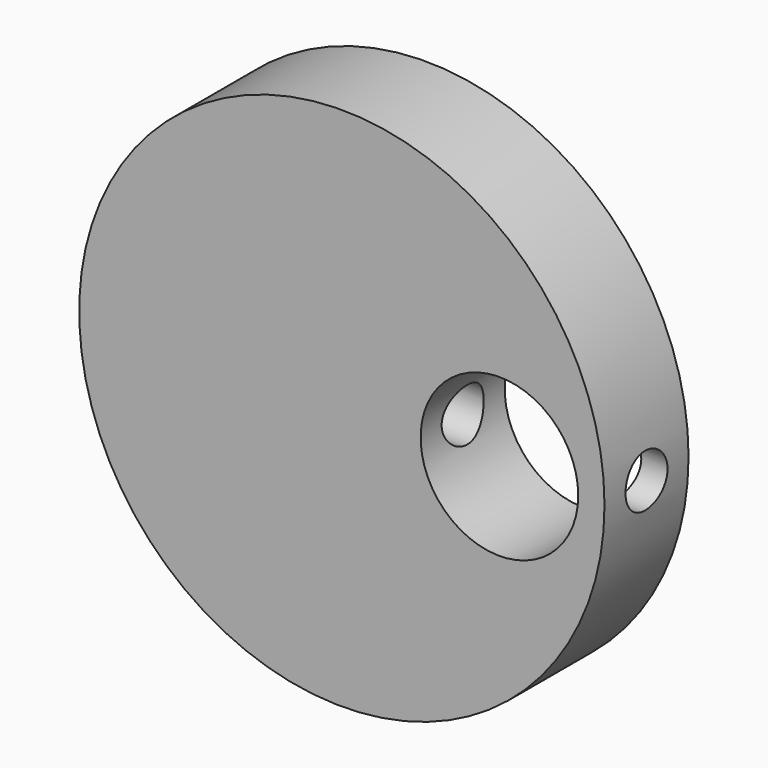
from build123d import *

# Parameters (mm, degrees)
F0_R     = 15.875
F0_R_2   = 4.7625
F1_DEPTH = 6.35
F3_D     = 3.175
F3_DEPTH = 15.876


with BuildPart() as f1:
    # F0 (on Front) → F1 (new body)
    with BuildSketch(Plane.XZ):
        Circle(F0_R)
        with Locations((9.525, 0)):
            Circle(F0_R_2, mode=Mode.SUBTRACT)
    extrude(amount=F1_DEPTH)

    # F3 (through all, one way)
    with BuildSketch(Plane(origin=(0, 0, 0), x_dir=(0, 1, 0), z_dir=(-1, 0, 0))):
        with Locations((-3.175, 0)):
            Circle(F3_D / 2)
    extrude(amount=-F3_DEPTH, mode=Mode.SUBTRACT)


solid = f1.part
